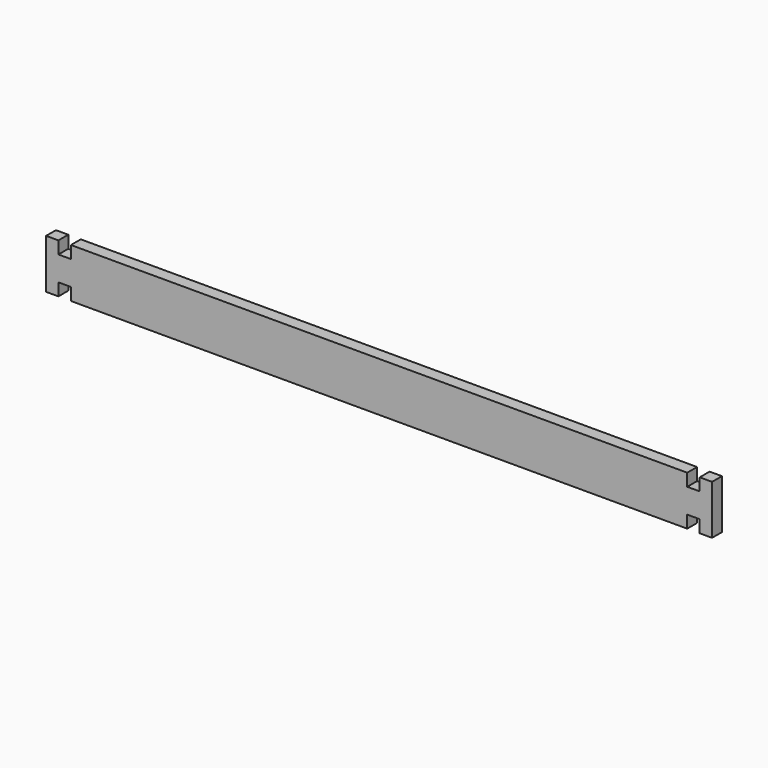
from build123d import *

# Parameters (mm, degrees)
F1_DEPTH = 3


# Not quite as in the source:
# - a feature names something its author has since deleted; it is built from what else it names


with BuildPart() as f1:
    # F0 (on Front) → F1 (new body)
    with BuildSketch(Plane.XZ):
        Polygon((-81.04, -2), (-78.04, -2), (-78.04, 1.02), (-75, 1.02), (-75, -2), (75, -2), (75, 1.02), (78.04, 1.02), (78.04, -2), (81.04, -2), (81.04, 10), (78.04, 10), (78.04, 6.98), (75, 6.98), (75, 10), (-75, 10), (-75, 6.98), (-78.04, 6.98), (-78.04, 10), (-81.04, 10), align=None)
    extrude(amount=F1_DEPTH)


solid = f1.part
